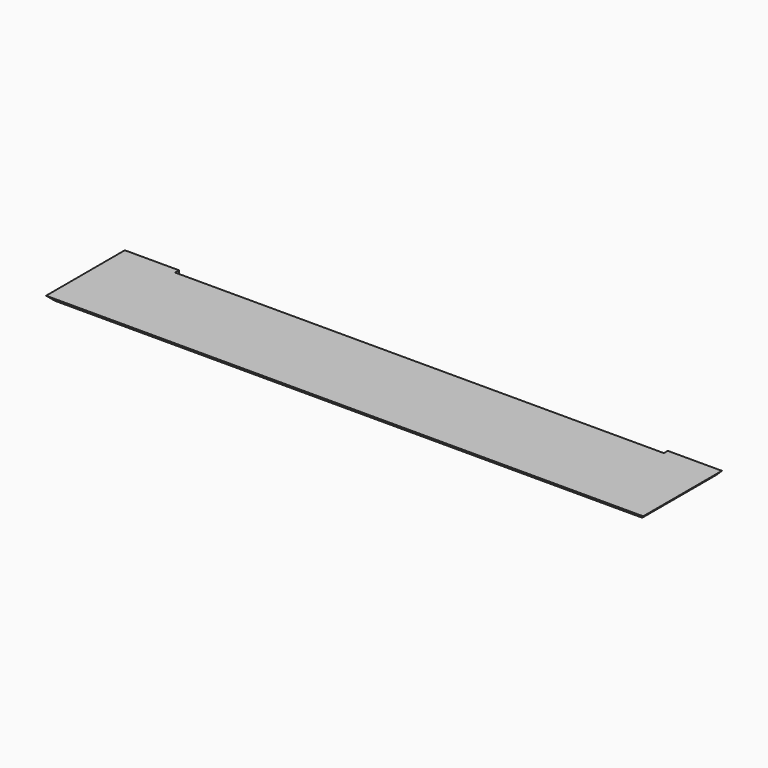
from build123d import *

# Parameters (mm, degrees)
F1_DEPTH = 19.05
F2_SIZE  = 19.04999


# Not quite as in the source:
# - a fillet or chamfer is up to 0.001 mm smaller than in the source, because OpenCascade refuses the exact size


with BuildPart() as f1:
    # F0 (on Top) → F1 (new body)
    with BuildSketch(Plane.XY):
        Polygon((-1155.7, -190.5), (1155.7, -190.5), (1155.7, 190.5), (946.15, 190.5), (946.15, 171.45), (-946.15, 171.45), (-946.15, 190.5), (-1155.7, 190.5), align=None)
    extrude(amount=F1_DEPTH)

    # F2 (size 19.05 in the source; OpenCascade refuses exactly that, so slightly less here)
    f2_edges = [f1.edges().sort_by_distance(p)[0] for p in [
        (-1155.7, 0, 0),
        (0, -190.5, 0),
        (1155.7, 0, 0),
    ]]
    chamfer(f2_edges, length=F2_SIZE)


solid = f1.part
